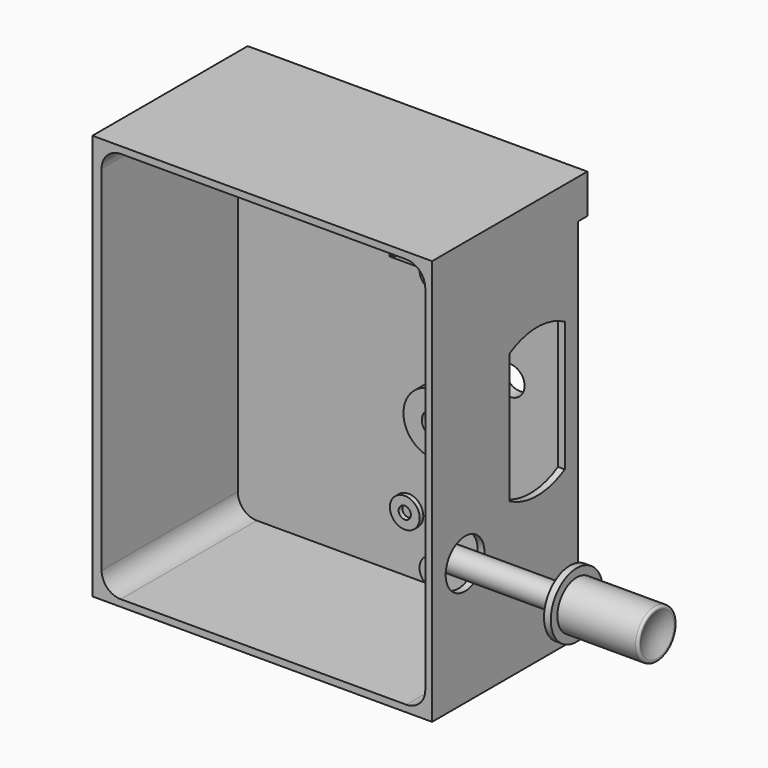
from build123d import *

# Parameters (mm, degrees)
F1_W      = 88.9
F1_H      = 106.172
F2_DEPTH  = 19.685
F3_W      = 88.9
F3_H      = 106.172
F4_DEPTH  = 31.115
F6_DEPTH  = 19.686
F8_R      = 6.35
F9_DEPTH  = 1.778
F12_DEPTH = 21.59
F13_R     = 1.5875
F13_R_2   = 3.2
F14_DEPTH = 3.275
F17_DEPTH = 2
F19_DEPTH = 3
F20_R     = 3.81
F20_R_2   = 1.5875
F21_DEPTH = 4
F24_R     = 0.6
F26_R     = 3.81
F26_R_2   = 1.65
F27_DEPTH = 18.796
F29_DEPTH = 16
F31_DEPTH = 3.2
F32_R     = 1.65
F33_DEPTH = 5.4
F34_R     = 0.6
F35_R     = 3.9
F35_R_2   = 1.6
F36_DEPTH = 1.2
F38_DEPTH = 5
F39_R     = 1.5
F40_DEPTH = 30
F41_R     = 0.6
F42_R     = 2.25
F43_DEPTH = 1
F44_R     = 2.4
F44_R_2   = 1.6
F45_DEPTH = 2.5


with BuildPart() as f2:
    # F1 (on Front) → F2 (new body)
    with BuildSketch(Plane.XZ):
        Rectangle(F1_W, F1_H)
    extrude(amount=F2_DEPTH)

    # F3 (on Front) → F4 (join)
    with BuildSketch(Plane.XZ):
        Rectangle(F3_W, F3_H)
    extrude(amount=-F4_DEPTH)

    # F5 (on Front) → F6 (cut, through all)
    with BuildSketch(Plane.XZ):
        with BuildLine():
            ThreePointArc((-37.044646, 51.308), (-40.5801799059, 49.8435339059), (-42.044646, 46.308))
            Line((-42.044646, 46.308), (-42.044646, -46.308))
            ThreePointArc((-42.044646, -46.308), (-40.5801799059, -49.8435339059), (-37.044646, -51.308))
            Line((-37.044646, -51.308), (37.672, -51.308))
            ThreePointArc((37.672, -51.308), (41.2075339059, -49.8435339059), (42.672, -46.308))
            Line((42.672, -46.308), (42.672, 46.308))
            ThreePointArc((42.672, 46.308), (41.2075339059, 49.8435339059), (37.672, 51.308))
            Line((37.672, 51.308), (-37.044646, 51.308))
        make_face()
    extrude(amount=F6_DEPTH, mode=Mode.SUBTRACT)

    # F8 (on face) → F9 (cut, through all)
    with BuildSketch(Plane.YZ.offset(44.45)):
        with Locations((-8.885, -21.006)):
            Circle(F8_R)
    extrude(amount=-F9_DEPTH, mode=Mode.SUBTRACT)

    # F11 (on offset) → F12 (cut)
    with BuildSketch(Plane.XZ.offset(-3.275)):
        with BuildLine():
            Line((37.672, 51.308), (-37.044646, 51.308))
            ThreePointArc((-37.044646, 51.308), (-40.5801799059, 49.8435339059), (-42.044646, 46.308))
            Line((-42.044646, 46.308), (-42.044646, -46.308))
            ThreePointArc((-42.044646, -46.308), (-40.5801799059, -49.8435339059), (-37.044646, -51.308))
            Line((-37.044646, -51.308), (37.672, -51.308))
            ThreePointArc((37.672, -51.308), (41.2075339059, -49.8435339059), (42.672, -46.308))
            Line((42.672, -46.308), (42.672, 46.308))
            ThreePointArc((42.672, 46.308), (41.2075339059, 49.8435339059), (37.672, 51.308))
        make_face()
    extrude(amount=-F12_DEPTH, mode=Mode.SUBTRACT)

    # F13 (on face) → F14 (cut, through all)
    with BuildSketch(Plane.XZ):
        with BuildLine():
            Line((29, 40.6241929313), (29, 51.308))
            Line((29, 51.308), (-37.044646, 51.308))
            ThreePointArc((-37.044646, 51.308), (-40.5801799059, 49.8435339059), (-42.044646, 46.308))
            Line((-42.044646, 46.308), (-42.044646, -46.308))
            ThreePointArc((-42.044646, -46.308), (-40.5801799059, -49.8435339059), (-37.044646, -51.308))
            Line((-37.044646, -51.308), (29, -51.308))
            Line((29, -51.308), (29, -35.5441929313))
            ThreePointArc((29, -35.5441929313), (25.41, -31.75), (29, -27.9558070687))
            Line((29, -27.9558070687), (29, -5.457243275))
            ThreePointArc((29, -5.457243275), (21.21, 2.54), (29, 10.537243275))
            Line((29, 10.537243275), (29, 33.0358070687))
            ThreePointArc((29, 33.0358070687), (25.41, 36.83), (29, 40.6241929313))
        make_face()
        with Locations((29.21, -31.75)):
            Circle(F13_R)
        with Locations((29.21, 36.83)):
            Circle(F13_R)
        with Locations((29.21, 2.54)):
            Circle(F13_R_2)
    extrude(amount=-F14_DEPTH, mode=Mode.SUBTRACT)

    # F16 (on face) → F17 (cut)
    with BuildSketch(Plane.YZ.offset(44.45)):
        with BuildLine():
            ThreePointArc((5.675, -12.544), (14.7, -14.9700032426), (23.725, -12.544))
            Line((23.725, -12.544), (23.725, 21.496))
            ThreePointArc((23.725, 21.496), (14.7, 23.9220032426), (5.675, 21.496))
            Line((5.675, 21.496), (5.675, -12.544))
        make_face()
    extrude(amount=-F17_DEPTH, mode=Mode.SUBTRACT)

    # F18 (on face) → F19 (cut)
    with BuildSketch(Plane(origin=(0, 31.115, 0), x_dir=(-1, 0, 0), z_dir=(0, 1, 0))):
        with BuildLine():
            Line((-25.21, 42.83), (-44.45, 42.83))
            Line((-44.45, 42.83), (-44.45, -37.75))
            Line((-44.45, -37.75), (-25.21, -37.75))
            ThreePointArc((-25.21, -37.75), (-19.5531457505, -35.4068542495), (-17.21, -29.75))
            Line((-17.21, -29.75), (-17.21, 34.83))
            ThreePointArc((-17.21, 34.83), (-19.5531457505, 40.4868542495), (-25.21, 42.83))
        make_face()
    extrude(amount=-F19_DEPTH, mode=Mode.SUBTRACT)

    # F20 (on face) → F21 (cut)
    with BuildSketch(Plane(origin=(0, 28.115, 0), x_dir=(-1, 0, 0), z_dir=(0, 1, 0))):
        with Locations((-29.21, 2.54)):
            Circle(F20_R)
        with Locations((-29.21, 36.83)):
            Circle(F20_R_2)
        with Locations((-29.21, -31.75)):
            Circle(F20_R_2)
    extrude(amount=-F21_DEPTH, mode=Mode.SUBTRACT)

    # F35 (on face) → F36 (join)
    with BuildSketch(Plane.XZ.offset(-24.865)):
        with Locations((2.616, -36.093)):
            Circle(F35_R)
        with Locations((2.616, -36.093)):
            Circle(F35_R_2, mode=Mode.SUBTRACT)
    extrude(amount=F36_DEPTH)

    # F44 (on face) → F45 (join)
    with BuildSketch(Plane.XZ.offset(-24.865)):
        with Locations((-36, 43.5)):
            Circle(F44_R)
        with Locations((-36, 43.5)):
            Circle(F44_R_2, mode=Mode.SUBTRACT)
        with Locations((-36, 28.5)):
            Circle(F44_R)
        with Locations((-36, 28.5)):
            Circle(F44_R_2, mode=Mode.SUBTRACT)
        with Locations((-12, 43.5)):
            Circle(F44_R)
        with Locations((-12, 43.5)):
            Circle(F44_R_2, mode=Mode.SUBTRACT)
        with Locations((-12, 28.5)):
            Circle(F44_R)
        with Locations((-12, 28.5)):
            Circle(F44_R_2, mode=Mode.SUBTRACT)
    extrude(amount=F45_DEPTH)


with BuildPart() as f23:
    # F22 (on offset) → F23 (revolve)
    with BuildSketch(Plane.XZ.offset(8.885)):
        with BuildLine():
            Line((38.9030366398, -17.831), (38.9030366398, -21.006))
            Line((38.9030366398, -21.006), (93.45, -21.006))
            ThreePointArc((93.45, -21.006), (93.8910398043, -17.7148787627), (95.1830366398, -14.656))
            Line((95.1830366398, -14.656), (73.6830366398, -14.656))
            Line((73.6830366398, -14.656), (73.6830366398, -12.506))
            Line((73.6830366398, -12.506), (71.9030366398, -12.506))
            Line((71.9030366398, -12.506), (71.9030366398, -17.831))
            Line((71.9030366398, -17.831), (38.9030366398, -17.831))
        make_face()
    revolve(axis=Axis((38.9030366398, -8.885, -21.006), (1, 0, 0)))

    # F24
    f24_edges = [f23.edges().sort_by_distance(p)[0] for p in [
        (95.183037, -8.885, -27.356),
        (93.89104, -8.885, -17.714879),
    ]]
    fillet(f24_edges, radius=F24_R)


with BuildPart() as f27:
    # F26 (on face) → F27 (new body)
    with BuildSketch(Plane(origin=(0, 3.275, 0), x_dir=(-1, 0, 0), z_dir=(0, 1, 0))):
        with Locations((-29.21, 36.83)):
            Circle(F26_R)
        with Locations((-29.21, 36.83)):
            Circle(F26_R_2, mode=Mode.SUBTRACT)
    extrude(amount=F27_DEPTH)

    # F28 (on face) → F29 (join)
    with BuildSketch(Plane(origin=(0, 3.275, 0), x_dir=(-1, 0, 0), z_dir=(0, 1, 0))):
        Polygon((-25.7686001944, 38.4648906319), (-25.7464839036, 35.2425), (-14.986, 35.2425), (-14.986, 38.4175), align=None)
    extrude(amount=F29_DEPTH)

    # F30 (on face) → F31 (join)
    with BuildSketch(Plane(origin=(0, 3.275, 0), x_dir=(-1, 0, 0), z_dir=(0, 1, 0))):
        with BuildLine():
            Line((-16.688, 38.4249804643), (-16.688, 40.615))
            ThreePointArc((-16.688, 40.615), (-19.8490456847, 43.7899693348), (-23.0378773399, 40.6429083611))
            Line((-23.0378773399, 40.6429083611), (-23.0378773399, 38.4528888253))
            Line((-23.0378773399, 38.4528888253), (-16.688, 38.4249804643))
        make_face()
    extrude(amount=F31_DEPTH)

    # F32 (on face) → F33 (join)
    with BuildSketch(Plane(origin=(0, 3.275, 0), x_dir=(-1, 0, 0), z_dir=(0, 1, 0))):
        with Locations((-19.863, 40.615)):
            Circle(F32_R)
    extrude(amount=-F33_DEPTH)

    # F34
    f34_edges = [f27.edges().sort_by_distance(p)[0] for p in [
        (21.513, -2.125, 40.615),
    ]]
    fillet(f34_edges, radius=F34_R)


with BuildPart() as f38:
    # F37 (on face) → F38 (new body)
    with BuildSketch(Plane(origin=(0, 3.275, 0), x_dir=(-1, 0, 0), z_dir=(0, 1, 0))):
        Polygon((-42.2148, -24.638), (-42.2148, -26.162), (-36.0934, -26.162), (-36.0934, -18.034), (-42.2148, -18.034), (-42.2148, -19.558), (-38.1254, -19.558), (-38.1254, -24.638), align=None)
    extrude(amount=F38_DEPTH)


with BuildPart() as f40:
    # F39 (on face) → F40 (new body)
    with BuildSketch(Plane(origin=(0, 28.115, 0), x_dir=(-1, 0, 0), z_dir=(0, 1, 0))):
        with Locations((-29.21, 36.83)):
            Circle(F39_R)
    extrude(amount=-F40_DEPTH)

    # F41
    f41_edges = [f40.edges().sort_by_distance(p)[0] for p in [
        (30.71, -1.885, 36.83),
    ]]
    fillet(f41_edges, radius=F41_R)

    # F42 (on face) → F43 (join)
    with BuildSketch(Plane(origin=(0, 28.115, 0), x_dir=(-1, 0, 0), z_dir=(0, 1, 0))):
        with Locations((-29.21, 36.83)):
            Circle(F42_R)
    extrude(amount=F43_DEPTH)


solid = Compound([f2.part, f23.part, f27.part, f38.part, f40.part])
